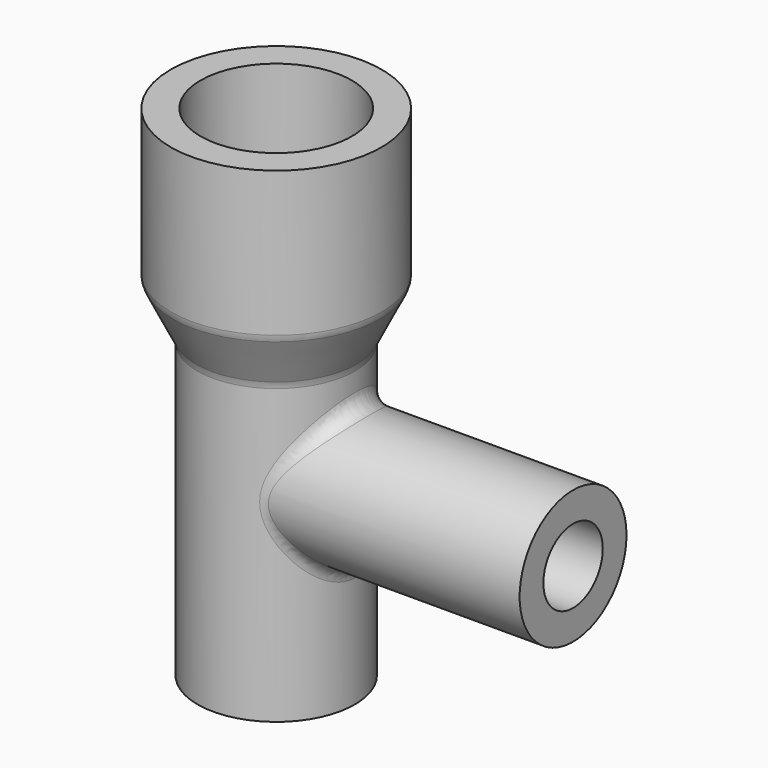
from build123d import *

# Parameters (mm, degrees)
F2_R     = 2.5
F3_REACH = 14.1720678119
F5_R     = 4.5
F5_R_2   = 2.5
F7_R     = 1


with BuildPart() as f1:
    # F0 (on Front) → F1 (revolve)
    with BuildSketch(Plane.XZ):
        Polygon((-5.3, 20), (-5.3, 0), (-3.3, 0), (-3.3, 20), (-5.1, 23.6349634528), (-5.1, 33.6349634528), (-7.1, 33.6349634528), (-7.1, 23.6349634528), align=None)
    revolve(axis=Axis((0, 0, 10.0998366252), (0, 0, 1)))

    f3_end = f1.faces().sort_by_distance((5.3, 0, 10))[0]
    # F2 (on Right) → F3 (cut, up to a face of the model that its end follows)
    with BuildSketch(Plane.YZ):
        with Locations((0, 13)):
            Circle(F2_R)
    f3_long = extrude(amount=F3_REACH, mode=Mode.PRIVATE)
    add(split(f3_long, bisect_by=f3_end, keep=Keep.BOTTOM, mode=Mode.PRIVATE), mode=Mode.SUBTRACT)

    # F5 (on offset) → F6 (join, up to the next surface of F1)
    with BuildSketch(Plane.YZ.offset(20)):
        with Locations((0, 13)):
            Circle(F5_R)
        with Locations((0, 13)):
            Circle(F5_R_2, mode=Mode.SUBTRACT)
    extrude(until=Until.NEXT, dir=(-1, 0, 0))

    # F7
    f7_edges = [f1.edges().sort_by_distance(p)[0] for p in [
        (5.3, 0, 20),
        (7.1, 0, 23.634963),
        (2.8, -4.5, 13),
        (5.1, 0, 23.634963),
        (3.3, 0, 20),
    ]]
    fillet(f7_edges, radius=F7_R)


solid = f1.part
